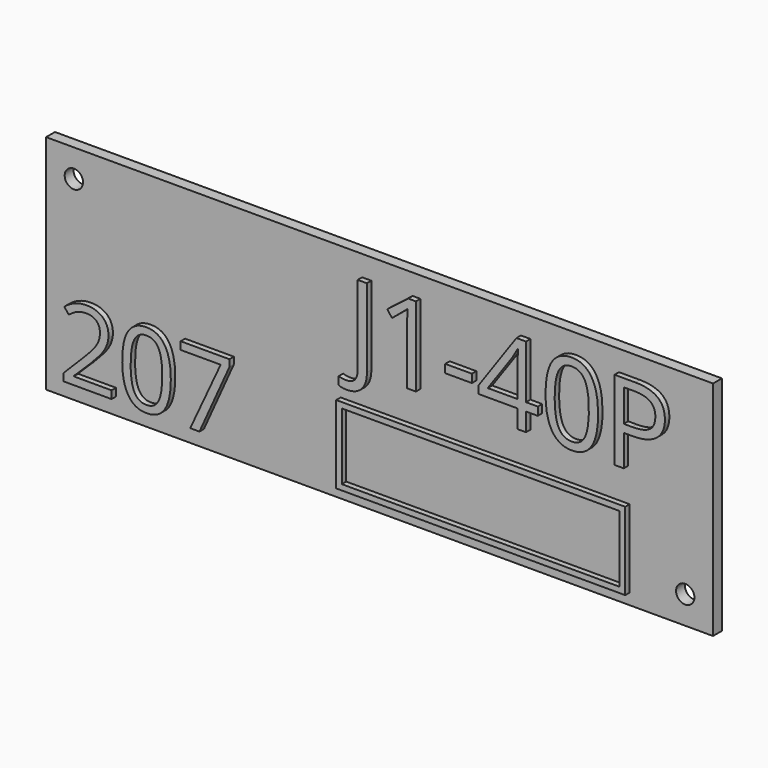
from build123d import *

# Parameters (mm, degrees)
F0_W         = 120
F0_H         = 40
F1_DEPTH     = 2
F3_D         = 3.3
F4_TEXT_SIZE = 20.0156372166
F5_DEPTH     = 1
F6_TEXT_SIZE = 18.5054667028
F7_DEPTH     = 1
F8_W         = 52
F8_H         = 14
F8_W_2       = 49.99999962
F8_H_2       = 11.99999962
F9_DEPTH     = 1


# Not quite as in the source:
# - Text() gives the source's letters only with a copy of the font that has no kerning and outlines rounded to 1/6400 em; it was checked with that copy


with BuildPart() as f1:
    # F0 (on Front) → F1 (new body)
    with BuildSketch(Plane.XZ):
        Rectangle(F0_W, F0_H)
    extrude(amount=F1_DEPTH)

    # F3 (through all)
    with Locations(Plane.XZ.offset(2)):
        with Locations((-55, 15), (55, -15)):
            Hole(F3_D / 2)

    # F4 (on face) → F5 (join)
    with BuildSketch(Plane.XZ.offset(2)):
        with Locations((-5, 2)):
            Text('J1-40P', F4_TEXT_SIZE, font='Open Sans', text_align=(TextAlign.LEFT, TextAlign.BOTTOM))
    extrude(amount=F5_DEPTH)

    # F6 (on face) → F7 (join)
    with BuildSketch(Plane.XZ.offset(2)):
        with Locations((-57, -17)):
            Text('207', F6_TEXT_SIZE, font='Open Sans', text_align=(TextAlign.LEFT, TextAlign.BOTTOM))
    extrude(amount=F7_DEPTH)

    # F8 (on face) → F9 (join)
    with BuildSketch(Plane.XZ.offset(2)):
        with Locations((19, -11)):
            Rectangle(F8_W, F8_H)
        with Locations((19, -11)):
            Rectangle(F8_W_2, F8_H_2, mode=Mode.SUBTRACT)
    extrude(amount=F9_DEPTH)


solid = f1.part
